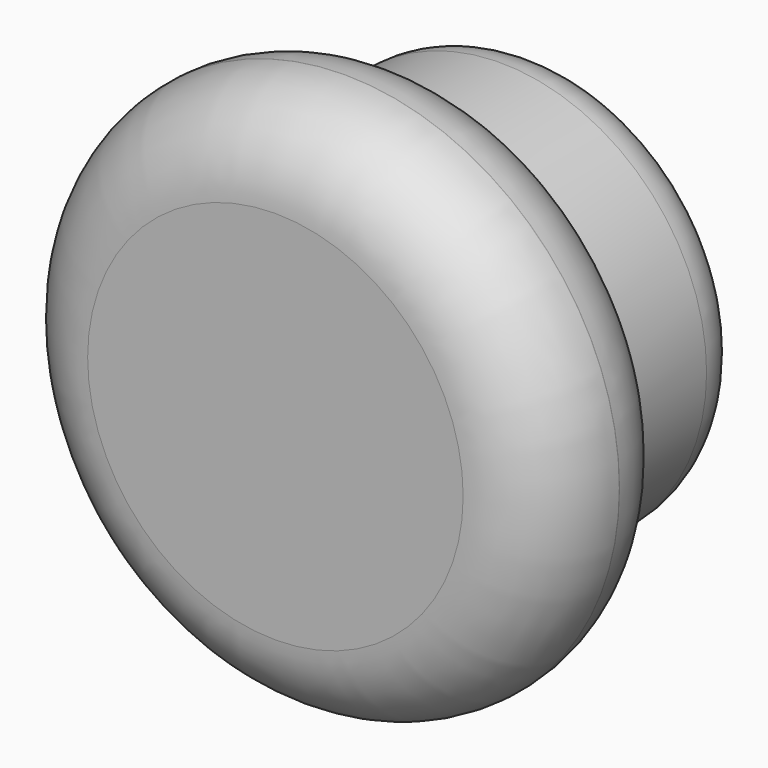
from build123d import *

# Parameters (mm, degrees)
F0_R     = 9.525
F1_DEPTH = 7.62
F2_R     = 12.7
F3_DEPTH = 7.9502
F5_R     = 2.54


# Not quite as in the source:
# - a fillet or chamfer that OpenCascade refuses, or shapes differently, is made with other operations: its cross-section is extruded or revolved along the edge and cut away or added


with BuildPart() as f1:
    # F0 (on Front) → F1 (new body)
    with BuildSketch(Plane.XZ):
        Circle(F0_R)
    extrude(amount=F1_DEPTH)

    # F2 (on face) → F3 (join)
    with BuildSketch(Plane.XZ.offset(7.62)):
        Circle(F2_R)
    extrude(amount=F3_DEPTH)

    # F4: fillet of radius 4.0132 on 2 edges, made by hand

    # F4_s1 → F4_t2 (revolve, cut)
    with BuildSketch(Plane.XY):
        with BuildLine():
            ThreePointArc((12.7, -11.557), (11.5245609343, -14.3947609343), (8.6868, -15.5702))
            Line((8.6868, -15.5702), (12.7, -15.5702))
            Line((12.7, -15.5702), (12.7, -11.557))
        make_face()
    revolve(axis=Axis((0, -15.5702, 0), (0, -1, 0)), mode=Mode.SUBTRACT)

    # F4_s3 → F4_t4 (revolve, cut)
    with BuildSketch(Plane.XY):
        with BuildLine():
            ThreePointArc((12.7, -11.5446904337), (11.8068671852, -9.0206153555), (9.525, -7.62))
            Line((9.525, -7.62), (12.7, -7.62))
            Line((12.7, -7.62), (12.7, -11.5446904337))
        make_face()
    revolve(axis=Axis((0, -7.62, 0), (0, -1, 0)), mode=Mode.SUBTRACT)

    # F5
    f5_edges = [f1.edges().sort_by_distance(p)[0] for p in [
        (-9.525, 0, 0),
    ]]
    fillet(f5_edges, radius=F5_R)


solid = f1.part
